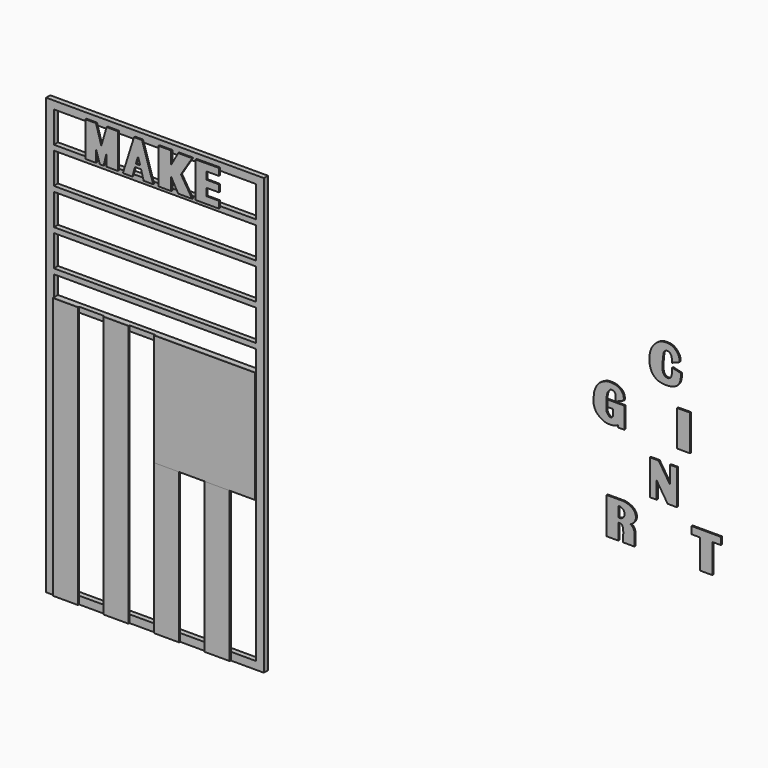
from build123d import *

# Parameters (mm, degrees)
F0_W     = 990.6
F0_H     = 25.4
F0_W_2   = 123.825
F0_W_3   = 495.3
F0_H_2   = 38.1
F1_DEPTH = 25.4
F2_W     = 495.3
F2_H     = 25.4
F3_DEPTH = 6.35
F2_W_2   = 123.825
F2_H_2   = 666.439058584
F2_H_3   = 38.1
F2_H_4   = 667.7452049673
F2_H_5   = 1221.0138589323
F4_W     = 123.825
F4_H     = 30.7621359825
F5_DEPTH = 6.35
F6_W     = 123.825
F6_H     = 29.4559895992
F7_DEPTH = 6.35
F9_DEPTH = 6.35


with BuildPart() as f1:
    # F0 (on Front) → F1 (new body)
    with BuildSketch(Plane.XZ):
        Polygon((409.575, 1067.611252743), (-657.225, 1067.611252743), (-657.225, -1065.988747257), (-619.125, -1065.988747257), (-619.125, -1027.888747257), (-619.125, 193.1251116753), (-619.125, 218.5251116753), (-619.125, 318.311252743), (-619.125, 343.711252743), (-619.125, 496.111252743), (-619.125, 521.511252743), (-619.125, 673.911252743), (-619.125, 699.311252743), (-619.125, 851.711252743), (-619.125, 877.111252743), (-619.125, 1029.511252743), (371.475, 1029.511252743), (371.475, 877.111252743), (371.475, 851.711252743), (371.475, 699.311252743), (371.475, 673.911252743), (371.475, 521.511252743), (371.475, 496.111252743), (371.475, 343.711252743), (371.475, 318.311252743), (371.475, 218.5251116753), (371.475, 193.1251116753), (371.475, -330.6875526905), (371.475, -1027.888747257), (371.475, -1065.988747257), (409.575, -1065.988747257), align=None)
        with Locations((-123.825, 864.411252743)):
            Rectangle(F0_W, F0_H)
        with Locations((-123.825, 686.611252743)):
            Rectangle(F0_W, F0_H)
        with Locations((-123.825, 508.811252743)):
            Rectangle(F0_W, F0_H)
        with Locations((-123.825, 331.011252743)):
            Rectangle(F0_W, F0_H)
        with Locations((-557.2125, 205.8251116753)):
            Rectangle(F0_W_2, F0_H)
        with Locations((-433.3875, 205.8251116753)):
            Rectangle(F0_W_2, F0_H)
        with Locations((-309.5625, 205.8251116753)):
            Rectangle(F0_W_2, F0_H)
        with Locations((-185.7375, 205.8251116753)):
            Rectangle(F0_W_2, F0_H)
        with Locations((123.825, 205.8251116753)):
            Rectangle(F0_W_3, F0_H)
        with Locations((309.5625, -1046.938747257)):
            Rectangle(F0_W_2, F0_H_2)
        with Locations((185.7375, -1046.938747257)):
            Rectangle(F0_W_2, F0_H_2)
        with Locations((61.9125, -1046.938747257)):
            Rectangle(F0_W_2, F0_H_2)
        with Locations((-61.9125, -1046.938747257)):
            Rectangle(F0_W_2, F0_H_2)
        with Locations((-185.7375, -1046.938747257)):
            Rectangle(F0_W_2, F0_H_2)
        with Locations((-309.5625, -1046.938747257)):
            Rectangle(F0_W_2, F0_H_2)
        with Locations((-433.3875, -1046.938747257)):
            Rectangle(F0_W_2, F0_H_2)
        with Locations((-557.2125, -1046.938747257)):
            Rectangle(F0_W_2, F0_H_2)
    extrude(amount=F1_DEPTH)


with BuildPart() as f3:
    # F2 (on face) → F3 (new body)
    with BuildSketch(Plane.XZ.offset(25.4)):
        Polygon((371.475, 193.1251116753), (-123.825, 193.1251116753), (-123.825, -330.6875526905), (0, -330.6875526905), (123.825, -330.6875526905), (247.65, -330.6875526905), (371.475, -330.6875526905), align=None)
        with Locations((123.825, 205.8251116753)):
            Rectangle(F2_W, F2_H)
    extrude(amount=F3_DEPTH)


with BuildPart() as f3b:
    # F2 (on face) → F3, piece 2 (new body)
    with BuildSketch(Plane.XZ.offset(25.4)):
        with Locations((-61.9125, -694.669217965)):
            Rectangle(F2_W_2, F2_H_2)
        with Locations((-61.9125, -1046.938747257)):
            Rectangle(F2_W_2, F2_H_3)
    extrude(amount=F3_DEPTH)

    # F4 (on face) → F5 (join)
    with BuildSketch(Plane.XZ.offset(31.75)):
        with Locations((-61.9125, -346.0686206818)):
            Rectangle(F4_W, F4_H)
    extrude(amount=-F5_DEPTH)


with BuildPart() as f3c:
    # F2 (on face) → F3, piece 3 (new body)
    with BuildSketch(Plane.XZ.offset(25.4)):
        with Locations((185.7375, -694.0161447734)):
            Rectangle(F2_W_2, F2_H_4)
        with Locations((185.7375, -1046.938747257)):
            Rectangle(F2_W_2, F2_H_3)
    extrude(amount=F3_DEPTH)

    # F6 (on face) → F7 (join)
    with BuildSketch(Plane.XZ.offset(31.75)):
        with Locations((185.7375, -345.4155474901)):
            Rectangle(F6_W, F6_H)
    extrude(amount=-F7_DEPTH)


with BuildPart() as f3d:
    # F2 (on face) → F3, piece 4 (new body)
    with BuildSketch(Plane.XZ.offset(25.4)):
        with Locations((-309.5625, 205.8251116753)):
            Rectangle(F2_W_2, F2_H)
        with Locations((-309.5625, -1046.938747257)):
            Rectangle(F2_W_2, F2_H_3)
        with Locations((-309.5625, -417.3818177909)):
            Rectangle(F2_W_2, F2_H_5)
    extrude(amount=F3_DEPTH)


with BuildPart() as f3e:
    # F2 (on face) → F3, piece 5 (new body)
    with BuildSketch(Plane.XZ.offset(25.4)):
        with Locations((-557.2125, -417.3818177909)):
            Rectangle(F2_W_2, F2_H_5)
        with Locations((-557.2125, -1046.938747257)):
            Rectangle(F2_W_2, F2_H_3)
        with Locations((-557.2125, 205.8251116753)):
            Rectangle(F2_W_2, F2_H)
    extrude(amount=F3_DEPTH)


with BuildPart() as f9:
    # F8 (on Front) → F9 (new body)
    with BuildSketch(Plane.XZ):
        Polygon((2091.6676521301, 464.614033699), (2039.3931865692, 464.614033699), (2039.3931865692, 293.6691343784), (2091.6676521301, 293.6691343784), (2091.6676521301, 354.4043004513), (2110.6436252594, 293.6691343784), (2129.1837692261, 293.6691343784), (2143.942117691, 354.4043004513), (2143.942117691, 293.6691343784), (2198.4474658966, 293.6691343784), (2198.4474658966, 464.614033699), (2143.942117691, 464.614033699), (2117.8050041199, 375.7970333099), align=None)
    extrude(amount=F9_DEPTH)


with BuildPart() as f9b:
    # F8 (on Front) → F9, piece 2 (new body)
    with BuildSketch(Plane.XZ):
        Polygon((1993.3441877365, 807.7932596207), (1938.853263855, 980.5018305779), (1899.6013402939, 980.5018305779), (1845.1104164124, 807.7932596207), (1891.7509317398, 807.7932596207), (1904.2191505432, 853.0484437943), (1919.2273020744, 853.0484437943), (1934.2354536057, 853.0484437943), (1946.7036724091, 807.7932596207), align=None)
        Polygon((1930.0793409348, 868.7492609024), (1919.2273020744, 868.7492609024), (1908.3752632141, 868.7492609024), (1919.2273020744, 902.9214978218), align=None, mode=Mode.SUBTRACT)
    extrude(amount=F9_DEPTH)


with BuildPart() as f9c:
    # F8 (on Front) → F9, piece 3 (new body)
    with BuildSketch(Plane.XZ):
        Polygon((2747.3881244659, 721.4146852493), (2685.3468418121, 721.4146852493), (2685.3468418121, 546.3929772377), (2747.3881244659, 546.3929772377), (2747.3881244659, 607.7812314034), (2781.3477516174, 546.3929772377), (2849.9195575714, 546.3929772377), (2795.0620651245, 633.9038312435), (2849.9195575714, 721.4146852493), (2781.3477516174, 721.4146852493), (2747.3881244659, 660.0264310837), align=None)
    extrude(amount=F9_DEPTH)


with BuildPart() as f9d:
    # F8 (on Front) → F9, piece 4 (new body)
    with BuildSketch(Plane.XZ):
        with BuildLine():
            Line((2155.350160224, 234.2979460955), (2073.7190246582, 234.2979460955))
            Line((2073.7190246582, 234.2979460955), (2073.7190246582, 56.0108609498))
            Line((2073.7190246582, 56.0108609498), (2131.8418979645, 56.0108609498))
            Line((2131.8418979645, 56.0108609498), (2131.8418979645, 134.3788057566))
            add(Edge.make_bspline(
                [(2131.8418979645, 134.3788057566), (2138.7055283526, 134.2567607872), (2159.2556202825, 134.0584523476), (2155.6730909061, 86.5738363862), (2153.3932685852, 56.0108609498)],
                knots=[0, 0, 0, 0, 0.3371338862, 1, 1, 1, 1], degree=3))
            Line((2153.3932685852, 56.0108609498), (2210.2098464966, 56.0108609498))
            Line((2210.2098464966, 56.0108609498), (2210.2098464966, 114.7868260741))
            ThreePointArc((2210.2098464966, 114.7868260741), (2204.9940914765, 133.0634792228), (2190.91796875, 145.8346545696))
            add(Edge.make_bspline(
                [(2155.350160224, 234.2979460955), (2161.5485353501, 234.2979460955), (2174.5294497989, 231.1672096161), (2197.7863726608, 222.4554276719), (2213.8241112218, 205.9997458241), (2219.90923869, 183.0343361995), (2210.8564132328, 158.3663775941), (2197.5011779614, 149.9731353096), (2190.91796875, 145.8346545696)],
                knots=[0, 0, 0, 0, 0.1538167235, 0.3275199284, 0.4925295763, 0.658734368, 0.8317817509, 1, 1, 1, 1], degree=3))
        make_face()
        with BuildLine():
            ThreePointArc((2131.8418979645, 205.3172141314), (2162.1408243863, 180.6677430868), (2131.8418979645, 156.0182720423))
            Line((2131.8418979645, 156.0182720423), (2131.8418979645, 205.3172141314))
        make_face(mode=Mode.SUBTRACT)
    extrude(amount=F9_DEPTH)


with BuildPart() as f9e:
    # F8 (on Front) → F9, piece 5 (new body)
    with BuildSketch(Plane.XZ):
        Polygon((2482.4001789093, 722.2290635109), (2419.5971488953, 721.7673063278), (2419.5971488953, 546.749830246), (2482.4001789093, 546.749830246), align=None)
    extrude(amount=F9_DEPTH)


with BuildPart() as f9f:
    # F8 (on Front) → F9, piece 6 (new body)
    with BuildSketch(Plane.XZ):
        with BuildLine():
            Line((2437.7918243408, 877.6104450226), (2395.307302475, 888.231575489))
            add(Edge.make_bspline(
                [(2393.4602737427, 908.0883860588), (2393.7721027151, 914.4281057242), (2394.3839280469, 926.8669790505), (2390.0271950755, 944.5131251735), (2375.7993138751, 953.7926058436), (2365.8800103622, 952.5216226385), (2351.6341579116, 945.0952973151), (2349.2959387939, 906.263361658), (2346.4035695109, 882.5147685977), (2348.6332296602, 847.0204995943), (2364.9613269648, 836.2489456382), (2379.5666019557, 835.355994476), (2390.5775933699, 844.3752426647), (2394.0904944558, 862.0728149407), (2394.8729861714, 878.8947072162), (2395.307302475, 888.231575489)],
                knots=[0, 0, 0, 0, 0.0765922848, 0.1502782109, 0.2190088175, 0.2725362013, 0.3371804117, 0.443000958, 0.5349859204, 0.6356768052, 0.7090668455, 0.7735014717, 0.835677906, 0.9087942236, 1, 1, 1, 1], degree=3))
            Line((2393.4602737427, 908.0883860588), (2429.479598999, 922.4038124084))
            add(Edge.make_bspline(
                [(2429.479598999, 922.4038124084), (2430.4856926929, 929.1040651384), (2432.7357763486, 944.0888814123), (2413.2267195364, 972.0078734025), (2389.5526908447, 987.0296602676), (2350.9768805067, 987.7565196429), (2323.0754687425, 976.8116229377), (2296.6190851977, 948.6395030679), (2284.6237299524, 917.8011334142), (2282.0679845549, 880.0493207353), (2288.4852626897, 843.1210754978), (2315.7214168686, 807.582588133), (2371.4426329997, 798.7715223048), (2424.348024326, 812.7223976968), (2438.3165031784, 850.9051567702), (2437.9572884871, 869.1885926332), (2437.7918243408, 877.6104450226)],
                knots=[0, 0, 0, 0, 0.0548950985, 0.1227704385, 0.1864419, 0.259202592, 0.3249862362, 0.3981482004, 0.4672516874, 0.5405478658, 0.6136640235, 0.6906985466, 0.7796889358, 0.8657806158, 0.9381748677, 1, 1, 1, 1], degree=3))
        make_face()
    extrude(amount=F9_DEPTH)


with BuildPart() as f9g:
    # F8 (on Front) → F9, piece 7 (new body)
    with BuildSketch(Plane.XZ):
        Polygon((2858.457326889, 981.4032316208), (2743.9339160919, 981.4032316208), (2743.9339160919, 894.1253721714), (2743.9339160919, 806.847512722), (2858.457326889, 806.847512722), (2858.457326889, 840.5579924583), (2798.4249591827, 840.5579924583), (2798.4249591827, 876.577436924), (2858.9191436768, 877.0391941071), (2858.9191436768, 894.1253721714), (2858.9191436768, 911.2115502357), (2798.4249591827, 911.6733074188), (2798.4249591827, 947.6927518845), (2858.457326889, 947.6927518845), align=None)
        Polygon((2858.457326889, 982.3268055916), (2743.9339160919, 981.4032316208), (2858.457326889, 981.4032316208), align=None)
    extrude(amount=F9_DEPTH)


with BuildPart() as f9h:
    # F8 (on Front) → F9, piece 8 (new body)
    with BuildSketch(Plane.XZ):
        Polygon((2633.7785720825, 235.6516177848), (2489.8090199435, 235.6516177848), (2489.8090199435, 199.962541461), (2532.4921607971, 199.962541461), (2532.4921607971, 56.9200358708), (2592.5137996674, 56.9200358708), (2592.5137996674, 199.962541461), (2633.7785720825, 199.962541461), align=None)
    extrude(amount=F9_DEPTH)


with BuildPart() as f9i:
    # F8 (on Front) → F9, piece 9 (new body)
    with BuildSketch(Plane.XZ):
        Polygon((2328.7951889221, 465.4275178909), (2285.6659889221, 465.4275178909), (2285.6659889221, 293.3340966702), (2319.4282054901, 293.3340966702), (2319.4282054901, 376.3328194618), (2372.8849887848, 293.3340966702), (2417.9012775421, 293.3340966702), (2417.9012775421, 465.4275178909), (2384.1276111786, 465.4275178909), (2384.1276111786, 380.5530965328), align=None)
    extrude(amount=F9_DEPTH)


with BuildPart() as f9j:
    # F8 (on Front) → F9, piece 10 (new body)
    with BuildSketch(Plane.XZ):
        with BuildLine():
            Line((2117.219209671, 651.3947844505), (2157.5462818146, 668.2758331299))
            add(Edge.make_bspline(
                [(2157.5462818146, 668.2758331299), (2158.0206616646, 674.9241547292), (2158.9821372525, 688.3990080945), (2148.526617136, 707.5049694263), (2128.5915607322, 721.1837094106), (2108.8502749307, 726.3212210344), (2079.1195995948, 727.4539678488), (2062.0268088373, 720.7706128607), (2038.8031944792, 708.9162307373), (2024.0236528815, 689.2900267854), (2012.8806039572, 665.0506389726), (2010.0405774316, 634.3325205939), (2008.4398951332, 599.9643235211), (2025.392954949, 569.6393782861), (2040.3393886251, 559.855493601), (2047.3501682281, 555.2662611008)],
                knots=[0, 0, 0, 0, 0.0679697722, 0.1377614937, 0.2114707279, 0.2815365706, 0.3634439808, 0.4296415797, 0.5062278822, 0.5817417789, 0.6598943583, 0.7448413013, 0.8344755908, 0.9223590606, 1, 1, 1, 1], degree=3))
            add(Edge.make_bspline(
                [(2047.3501682281, 555.2662611008), (2054.2151067356, 551.5824010073), (2067.7244726247, 544.3330113977), (2088.8039985208, 543.1446523665), (2115.4833902848, 544.2868873398), (2126.0136090966, 551.826436005), (2130.8178901672, 555.2662611008)],
                knots=[0, 0, 0, 0, 0.2540986277, 0.5000352632, 0.771897321, 1, 1, 1, 1], degree=3))
            Line((2130.8178901672, 555.2662611008), (2130.8178901672, 543.543279171))
            Line((2130.8178901672, 543.543279171), (2160.3598594666, 543.543279171))
            Line((2160.3598594666, 543.543279171), (2160.3598594666, 647.6433873177))
            Line((2160.3598594666, 647.6433873177), (2078.2988071442, 647.6433873177))
            Line((2078.2988071442, 647.6433873177), (2078.2988071442, 615.2879595757))
            Line((2078.2988071442, 615.2879595757), (2105.4961681366, 615.2879595757))
            Line((2105.4961681366, 615.2879595757), (2105.4961681366, 585.2771401405))
            add(Edge.make_bspline(
                [(2117.219209671, 683.7502121925), (2115.7785045243, 686.9523744552), (2112.9592888138, 693.2184630987), (2103.577165491, 696.0257930087), (2090.8555179607, 695.9065361431), (2081.4279963178, 683.5267026639), (2075.4281865299, 671.8657669859), (2072.7688429299, 648.6521766039), (2072.4212583627, 630.0906336298), (2073.5579947404, 610.9521147793), (2072.2771857172, 593.8748620014), (2080.3608168965, 583.9173699257), (2087.956242717, 576.1288341752), (2095.8911613195, 574.7492959005), (2102.5356767028, 580.3765747468), (2104.5673027046, 583.7395691348), (2105.4961681366, 585.2771401405)],
                knots=[0, 0, 0, 0, 0.0638217385, 0.1248883218, 0.194615344, 0.2712475381, 0.3456062419, 0.4423856888, 0.5313743053, 0.6203629219, 0.7026373823, 0.7735960035, 0.8397597648, 0.8938150007, 0.9514519035, 1, 1, 1, 1], degree=3))
            Line((2117.219209671, 683.7502121925), (2117.219209671, 651.3947844505))
        make_face()
    extrude(amount=F9_DEPTH)


with BuildPart() as f9_1:
    # F10: moved
    add(f9.part.moved(Location((-2499.36, -25.4, 576.58))))


with BuildPart() as f9b_1:
    # F11: moved
    add(f9b.part.moved(Location((-2120.9, -25.4, 60.96))))


with BuildPart() as f9c_1:
    # F12: moved
    add(f9c.part.moved(Location((-2786.38, -25.4, 320.04))))


with BuildPart() as f9g_1:
    # F13: moved
    add(f9g.part.moved(Location((-2664.46, -25.4, 58.42))))


with BuildPart() as f9c_2:
    # F14: moved
    add(f9c_1.part.moved(Location((0, 0, 3.81))))


with BuildPart() as f9c_3:
    # F15: moved
    add(f9c_2.part.moved(Location((0, 0, -2.032))))


with BuildPart() as f9g_2:
    # F16: moved
    add(f9g_1.part.moved(Location((0, 0, 3.302))))


solid = Compound([f1.part, f3.part, f3b.part, f3c.part, f3d.part, f3e.part, f9d.part, f9e.part, f9f.part, f9h.part, f9i.part, f9j.part, f9_1.part, f9b_1.part, f9c_3.part, f9g_2.part])
